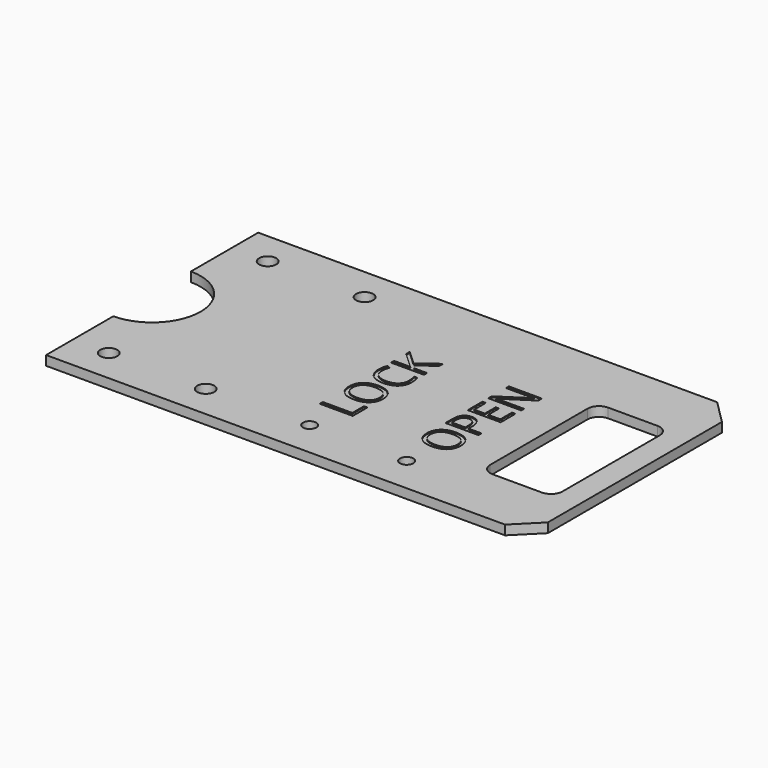
from build123d import *

# Parameters (mm, degrees)
F0_R         = 9
F1_DEPTH     = 10
F2_SIZE      = 25
F3_R         = 7
F4_DEPTH     = 10
F5_TEXT_SIZE = 48.6111111111
F6_DEPTH     = 1


# Not quite as in the source:
# - Text() gives the source's letters only with a copy of the font that has no kerning and outlines rounded to 1/6400 em; it was checked with that copy


with BuildPart() as f1:
    # F0 (on Top) → F1 (new body)
    with BuildSketch(Plane.XY):
        with BuildLine():
            Line((0, 88.5), (0, 0))
            Line((0, 0), (508, 0))
            Line((508, 0), (508, 279))
            Line((508, 279), (0, 279))
            Line((0, 279), (0, 190.5))
            ThreePointArc((0, 190.5), (51, 139.5), (0, 88.5))
        make_face()
        with Locations((38, 35)):
            Circle(F0_R, mode=Mode.SUBTRACT)
        with Locations((140, 35)):
            Circle(F0_R, mode=Mode.SUBTRACT)
        with Locations((38, 244)):
            Circle(F0_R, mode=Mode.SUBTRACT)
        with Locations((140, 244)):
            Circle(F0_R, mode=Mode.SUBTRACT)
        with BuildLine():
            Line((483, 203.5), (483, 75.5))
            ThreePointArc((483, 75.5), (479.4852813742, 67.0147186258), (471, 63.5))
            Line((471, 63.5), (419, 63.5))
            ThreePointArc((419, 63.5), (410.5147186258, 67.0147186258), (407, 75.5))
            Line((407, 75.5), (407, 203.5))
            ThreePointArc((407, 203.5), (410.5147186258, 211.9852813742), (419, 215.5))
            Line((419, 215.5), (471, 215.5))
            ThreePointArc((471, 215.5), (479.4852813742, 211.9852813742), (483, 203.5))
        make_face(mode=Mode.SUBTRACT)
    extrude(amount=F1_DEPTH)

    # F2
    f2_edges = [f1.edges().sort_by_distance(p)[0] for p in [
        (508, 0, 5),
        (508, 279, 5),
    ]]
    chamfer(f2_edges, length=F2_SIZE)

    # F3 (on face) → F4 (cut, through all)
    with BuildSketch(Plane.XY.offset(10)):
        with Locations((247, 38)):
            Circle(F3_R)
        with Locations((349, 38)):
            Circle(F3_R)
    extrude(amount=-F4_DEPTH, mode=Mode.SUBTRACT)

    # F5 (on face) → F6 (cut)
    with BuildSketch(Plane.XY.offset(10)):
        with Locations(Location((264.5, 68), (0, 0, 90))):
            Text('LOCK', F5_TEXT_SIZE, font='Open Sans', text_align=(TextAlign.LEFT, TextAlign.BOTTOM))
        with Locations(Location((366.5, 68), (0, 0, 90))):
            Text('OPEN', F5_TEXT_SIZE, font='Open Sans', text_align=(TextAlign.LEFT, TextAlign.BOTTOM))
    extrude(amount=-F6_DEPTH, mode=Mode.SUBTRACT)


solid = f1.part
